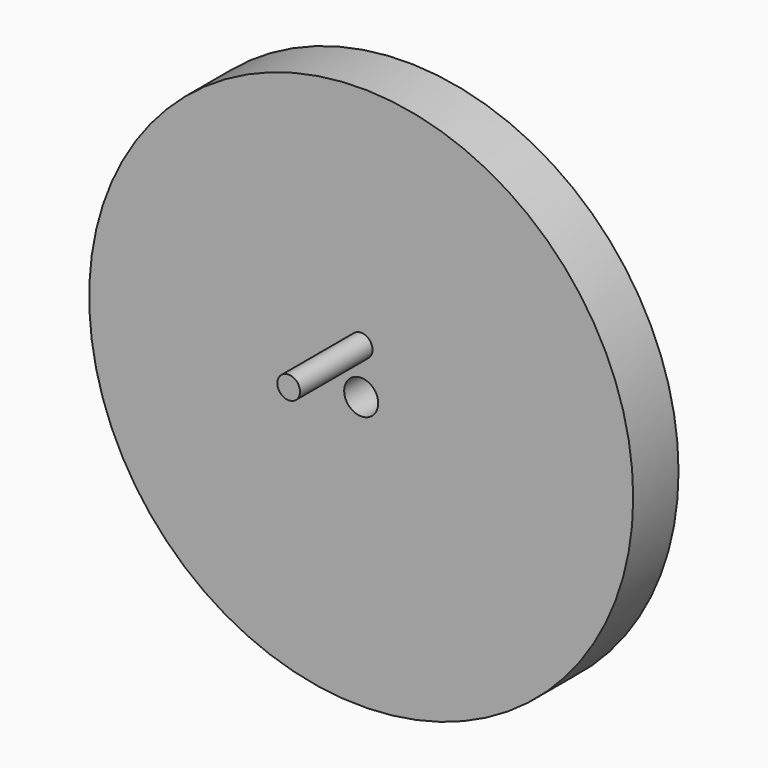
from build123d import *

# Parameters (mm, degrees)
F0_R          = 24
F0_R_2        = 8
F1_DEPTH      = 5
F2_DEPTH      = 11
F3_R          = 2.5
F4_DEPTH      = 0.5
F5_R          = 1.5
F6_DEPTH      = 25
F5_R_2        = 1
F7_DEPTH      = 8
F8_R          = 1.5
F9_DEPTH      = 24.001
F9_DEPTH_BACK = 24.001


with BuildPart() as f1:
    # F0 (on Front) → F1 (new body)
    with BuildSketch(Plane.XZ):
        Circle(F0_R)
        Circle(F0_R_2, mode=Mode.SUBTRACT)
        Circle(F0_R_2)
    extrude(amount=F1_DEPTH)

    # F0 (on Front) → F2 (join)
    with BuildSketch(Plane.XZ):
        Circle(F0_R_2)
    extrude(amount=-F2_DEPTH)

    # F3 (on face) → F4 (join)
    with BuildSketch(Plane(origin=(0, 11, 0), x_dir=(-1, 0, 0), z_dir=(0, 1, 0))):
        Circle(F3_R)
    extrude(amount=F4_DEPTH)

    # F5 (on face) → F6 (cut)
    with BuildSketch(Plane.XZ.offset(5)):
        Circle(F5_R)
    extrude(amount=-F6_DEPTH, mode=Mode.SUBTRACT)

    # F5 (on face) → F7 (join)
    with BuildSketch(Plane.XZ.offset(5)):
        with Locations((0, 4)):
            Circle(F5_R_2)
    extrude(amount=F7_DEPTH)

    # F8 (on Right) → F9 (cut, two sides)
    with BuildSketch(Plane.YZ) as f9_sk:
        with Locations((7, 0)):
            Circle(F8_R)
    extrude(amount=-F9_DEPTH, mode=Mode.SUBTRACT)
    extrude(f9_sk.sketch, amount=F9_DEPTH_BACK, mode=Mode.SUBTRACT)


solid = f1.part
